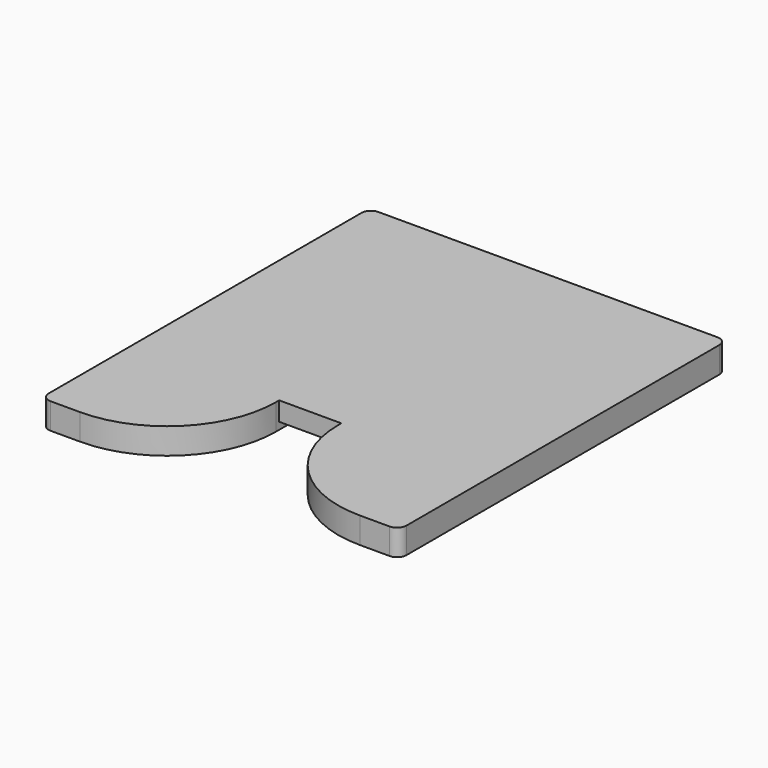
from build123d import *

# Parameters (mm, degrees)
F0_W     = 69.85
F0_H     = 80.01
F1_DEPTH = 5.08
F3_DEPTH = 1.397
F4_R     = 1
F5_R     = 1
F6_DEPTH = 1.397
F6_TAPER = -8
F7_W     = 12.1412
F7_H     = 22
F8_DEPTH = 3.684
F9_R     = 1.8396307345
F10_R    = 2.0944308897
F11_R    = 21.2450793489


with BuildPart() as f1:
    # F0 (on Top) → F1 (new body)
    with BuildSketch(Plane.XY):
        Rectangle(F0_W, F0_H)
    extrude(amount=F1_DEPTH)

    # F2 (on Top) → F3 (cut)
    with BuildSketch(Plane.XY):
        with BuildLine():
            ThreePointArc((6.0706, 15.0231522067), (0, 21.0937522067), (-6.0706, 15.0231522067))
            Line((-6.0706, 15.0231522067), (-6.0706, -3.937))
            Line((-6.0706, -3.937), (-6.0706, -8.7576295534))
            ThreePointArc((-6.0706, -8.7576295534), (-4.662, -10.9752828266), (-6.0706, -13.1929360997))
            Line((-6.0706, -13.1929360997), (-6.0706, -17.907))
            Line((-6.0706, -17.907), (-6.0706, -40.7645274005))
            Line((-6.0706, -40.7645274005), (6.0706, -40.7645274005))
            Line((6.0706, -40.7645274005), (6.0706, -13.1929360997))
            ThreePointArc((6.0706, -13.1929360997), (4.662, -10.9752828266), (6.0706, -8.7576295534))
            Line((6.0706, -8.7576295534), (6.0706, -3.937))
            Line((6.0706, -3.937), (6.0706, 15.0231522067))
        make_face()
    extrude(amount=F3_DEPTH, mode=Mode.SUBTRACT)

    # F4
    f4_edges = [f1.edges().sort_by_distance(p)[0] for p in [
        (-6.0706, -13.192936, 0.6985),
        (6.0706, -13.192936, 0.6985),
    ]]
    fillet(f4_edges, radius=F4_R)

    # F5 (on face) → F6 (join, through all)
    with BuildSketch(Plane(origin=(0, 0, 0), x_dir=(1, 0, 0), z_dir=(0, 0, -1))):
        with Locations((0, -15.171)):
            Circle(F5_R)
    extrude(amount=-F6_DEPTH, taper=F6_TAPER)

    # F7 (on face) → F8 (cut, through all)
    with BuildSketch(Plane(origin=(0, 0, 1.397), x_dir=(1, 0, 0), z_dir=(0, 0, -1))):
        with Locations((0, 29.005)):
            Rectangle(F7_W, F7_H)
    extrude(amount=-F8_DEPTH, mode=Mode.SUBTRACT)

    # F9
    f9_edges = [f1.edges().sort_by_distance(p)[0] for p in [
        (34.925, -40.005, 2.54),
        (-34.925, -40.005, 2.54),
        (-34.925, 40.005, 2.54),
        (34.925, 40.005, 2.54),
    ]]
    fillet(f9_edges, radius=F9_R)

    # F10
    f10_edges = [f1.edges().sort_by_distance(p)[0] for p in [
        (6.0706, -8.75763, 0.6985),
        (-6.0706, -8.75763, 0.6985),
    ]]
    fillet(f10_edges, radius=F10_R)

    # F11
    f11_edges = [f1.edges().sort_by_distance(p)[0] for p in [
        (6.0706, -40.005, 2.54),
        (-6.0706, -40.005, 2.54),
    ]]
    fillet(f11_edges, radius=F11_R)


solid = f1.part
